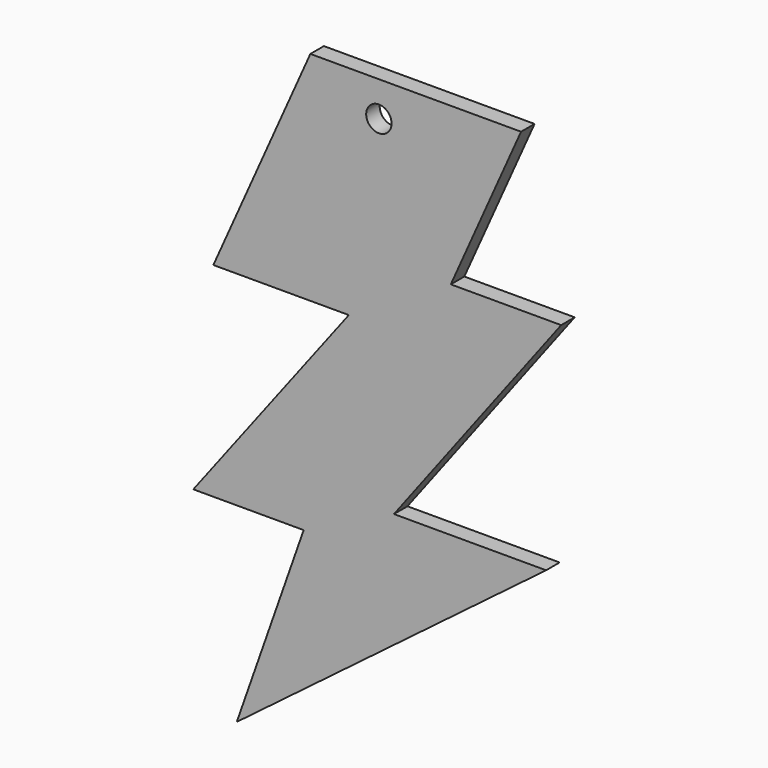
from build123d import *

# Parameters (mm, degrees)
F0_R     = 1.905
F1_DEPTH = 2.54
F2_DEPTH = 152


# Not quite as in the source:
# - an extrude ends at something that could not be found from the text; its depth is read off the source's solid


with BuildPart() as f1:
    # F0 (on Front) → F1 (new body)
    with BuildSketch(Plane.XZ):
        Polygon((-10.5372872204, 53.1882047653), (0, 76.7774991782), (-31.6092483094, 76.7774991782), (-46.1633428931, 44.156242162), (-25.8414391428, 44.156242162), (-49.1739995778, 13.5479401797), (-32.6154083014, 13.5479401797), (-42.6509156823, -15.0532610714), (3.763313638, 20.0710203499), (-19.0674699843, 20.0710203499), (6.0213026591, 53.1882047653), align=None)
        with Locations((-21.3299991501, 71.5437866839)):
            Circle(F0_R, mode=Mode.SUBTRACT)
    extrude(amount=F1_DEPTH)

    # F0 (on Front) → F2 (cut, through all)
    with BuildSketch(Plane.XZ):
        with Locations((-21.3299991501, 71.5437866839)):
            Circle(F0_R)
    extrude(amount=-F2_DEPTH, mode=Mode.SUBTRACT)


solid = f1.part
